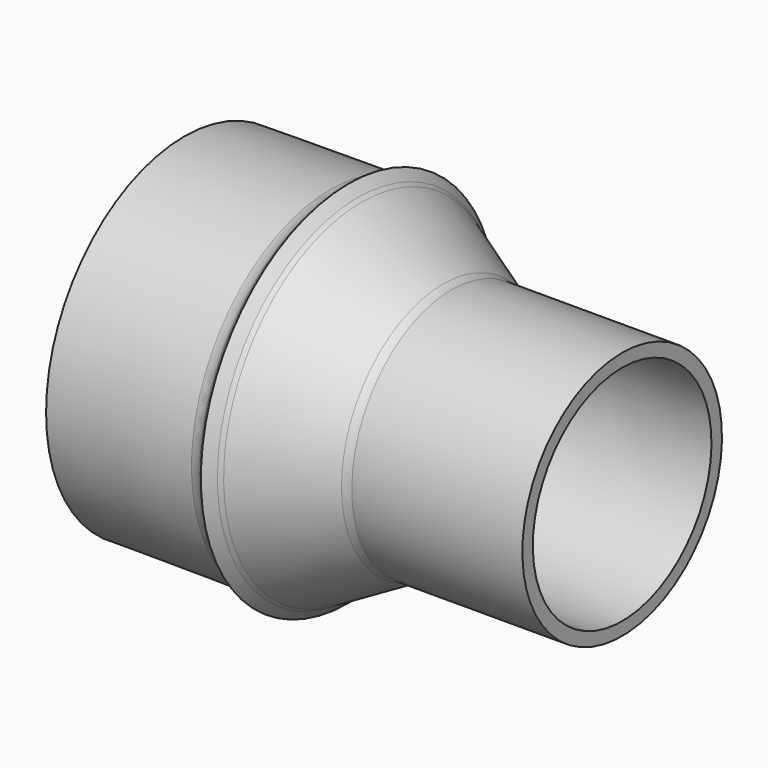
from build123d import *

# Parameters (mm, degrees)
F3_R = 5.08


# Not quite as in the source:
# - a variable given as a bare number and used for a length is read in inches; the dataset says mm whatever the document's units were


with BuildPart() as f2:
    # F1 (on Front) → F2 (revolve)
    with BuildSketch(Plane.XZ):
        Polygon((-25.4, 46.355), (0, 31.6153030303), (50.8, 32.385), (50.8, 36.195), (0, 36.195), (-25.4, 50.38725), (-28.575, 53.56225), (-31.75, 50.38725), (-76.2, 50.165), (-76.2, 46.355), align=None)
    revolve(axis=Axis((-24.3991323134, 0, 0), (-1, 0, 0)))

    # F3
    f3_edges = [f2.edges().sort_by_distance(p)[0] for p in [
        (-25.4, 0, -46.355),
        (0, 0, -31.615303),
        (0, 0, -36.195),
        (-31.75, 0, -50.38725),
        (-25.4, 0, -50.38725),
    ]]
    fillet(f3_edges, radius=F3_R)


solid = f2.part
